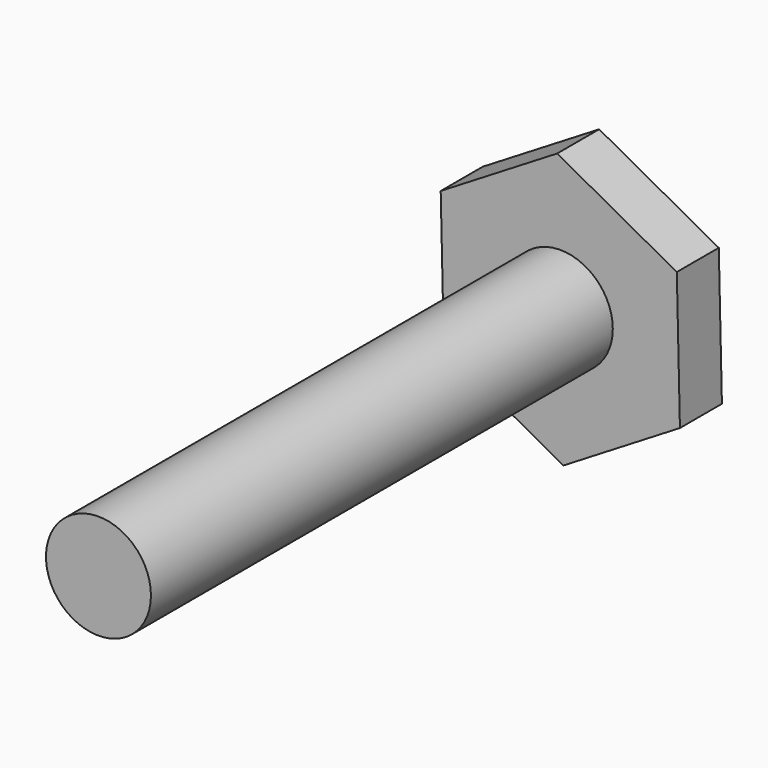
from build123d import *

# Parameters (mm, degrees)
F0_R     = 6.35
F1_DEPTH = 69.85
F2_R     = 6.35
F3_DEPTH = 6.35


with BuildPart() as f1:
    # F0 (on Front) → F1 (new body)
    with BuildSketch(Plane.XZ):
        Circle(F0_R)
    extrude(amount=F1_DEPTH)

    # F2 (on face) → F3 (join)
    with BuildSketch(Plane(origin=(0, 0, 0), x_dir=(-1, 0, 0), z_dir=(0, 1, 0))):
        Polygon((14.4728282073, 7.9192246264), (0.3781643989, 16.4934492053), (-14.0946638083, 8.5742245789), (-14.4728282073, -7.9192246264), (-0.3781643989, -16.4934492053), (14.0946638083, -8.5742245789), align=None)
        Circle(F2_R, mode=Mode.SUBTRACT)
        Circle(F2_R)
    extrude(amount=F3_DEPTH)


solid = f1.part
